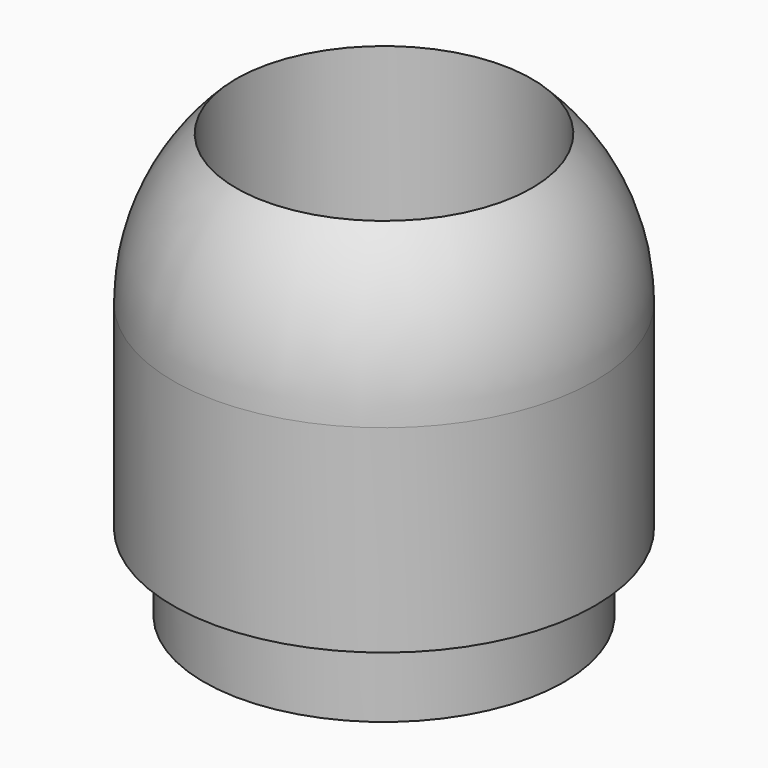
from build123d import *

# Parameters (mm, degrees)
F0_R     = 7
F0_R_2   = 5.8
F1_DEPTH = 3
F2_R     = 8.2
F3_DEPTH = 13.5
F4_R     = 5.75
F5_DEPTH = 16.501


# Not quite as in the source:
# - a fillet or chamfer that OpenCascade refuses, or shapes differently, is made with other operations: its cross-section is extruded or revolved along the edge and cut away or added


with BuildPart() as f1:
    # F0 (on Top) → F1 (new body)
    with BuildSketch(Plane.XY):
        Circle(F0_R)
        Circle(F0_R_2, mode=Mode.SUBTRACT)
    extrude(amount=F1_DEPTH)

    # F2 (on face) → F3 (join)
    with BuildSketch(Plane.XY.offset(3)):
        Circle(F2_R)
    extrude(amount=F3_DEPTH)

    # F4 (on face) → F5 (cut, through all)
    with BuildSketch(Plane.XY.offset(16.5)):
        Circle(F4_R)
    extrude(amount=-F5_DEPTH, mode=Mode.SUBTRACT)

    # F6: fillet of radius 8.1 on 1 edges, made by hand

    # F6_s1 → F6_t2 (revolve, cut)
    with BuildSketch(Plane.XZ):
        with BuildLine():
            ThreePointArc((8.2, 10.6959066169), (7.5624057783, 13.8459066169), (5.75, 16.5))
            Line((5.75, 16.5), (8.2, 16.5))
            Line((8.2, 16.5), (8.2, 10.6959066169))
        make_face()
    revolve(axis=Axis((0, 0, 16.5), (0, 0, 1)), mode=Mode.SUBTRACT)


solid = f1.part
